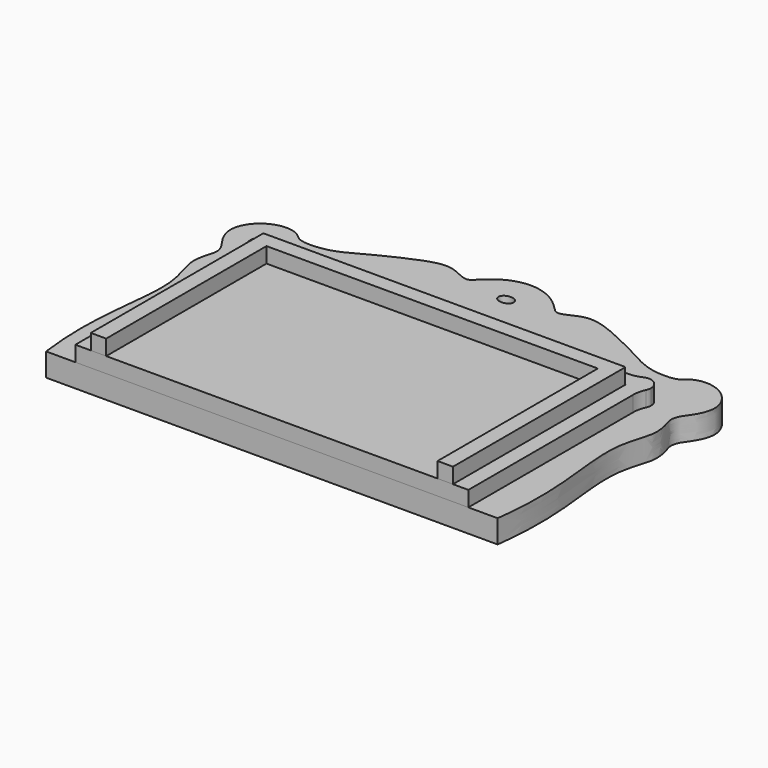
from build123d import *

# Parameters (mm, degrees)
F3_DEPTH  = 15
F5_DEPTH  = 10
F6_R      = 20
F8_DEPTH  = 10
F9_W      = 215
F9_H      = 130
F10_DEPTH = 10


# Not quite as in the source:
# - a feature names something its author has since deleted; it is built from what else it names


with BuildPart() as f3:
    # F2 (on offset) → F3 (new body)
    with BuildSketch(Plane.XY.offset(100)):
        with BuildLine():
            add(Edge.make_bspline(
                [(-146.497, 0), (-149.5984924285, 24.1158641447), (-148.0861706874, 57.3285451295), (-141.9737942158, 98.5465216918), (-150.8716245384, 120.1352309784), (-150.0828583406, 127.8333799004), (-149.2091995607, 133.0357574413), (-146.7644359487, 138.969514697), (-148.7060186985, 145.4416060002), (-153.4320405507, 150.8180485227), (-159.2044434643, 163.229297572), (-152.2232789146, 177.3369452319), (-138.5120912335, 183.3796622376), (-127.657061459, 180.8243319765), (-123.7549340061, 175.7598872143), (-115.4966109213, 174.5749138288), (-101.1868476342, 175.8719474345), (-83.9780063011, 186.2524528593), (-68.1221038647, 193.6100878861), (-57.6143130787, 198.1949467154), (-46.4912789312, 200.9893875839), (-38.3855377787, 198.1650207363), (-34.3252044535, 195.9531038256), (-28.5769681871, 194.0801714579), (-24.8215233637, 198.3952390386), (-15.2356704617, 207.2522812764), (0, 211.4399134414), (15.2356704617, 207.2522812764), (24.8215233637, 198.3952390386), (28.5769681871, 194.0801714579), (34.3252044535, 195.9531038256), (38.3855377787, 198.1650207363), (46.4912789312, 200.9893875839), (57.6143130787, 198.1949467154), (68.1221038647, 193.6100878861), (83.9780063011, 186.2524528593), (101.1868476342, 175.8719474345), (115.4966109213, 174.5749138288), (123.7549340061, 175.7598872143), (127.657061459, 180.8243319765), (138.5120912335, 183.3796622376), (152.2232789146, 177.3369452319), (159.2044434643, 163.229297572), (153.4320405507, 150.8180485227), (148.7060186985, 145.4416060002), (146.7644359487, 138.969514697), (149.2091995607, 133.0357574413), (150.0828583406, 127.8333799004), (150.8716245384, 120.1352309784), (141.9737942158, 98.5465216918), (148.0861706874, 57.3285451295), (149.5984924285, 24.1158641447), (146.497, 0)],
                knots=[0, 0, 0, 0, 0.0445117001, 0.0808774056, 0.107575939, 0.1227793119, 0.1357551155, 0.1500456603, 0.1643362052, 0.1797671231, 0.2002043009, 0.2219477978, 0.2436912948, 0.2620418522, 0.2758571435, 0.2916470183, 0.3132257177, 0.3392061483, 0.3632884541, 0.3827866647, 0.4019539182, 0.4183166408, 0.4309215947, 0.4439460967, 0.456795292, 0.4773590218, 0.5, 0.5226409782, 0.543204708, 0.5560539033, 0.5690784053, 0.5816833592, 0.5980460818, 0.6172133353, 0.6367115459, 0.6607938517, 0.6867742823, 0.7083529817, 0.7241428565, 0.7379581478, 0.7563087052, 0.7780522022, 0.7997956991, 0.8202328769, 0.8356637948, 0.8499543397, 0.8642448845, 0.8772206881, 0.892424061, 0.9191225944, 0.9554882999, 1, 1, 1, 1], degree=3))
            Line((-146.497, 0), (146.497, 0))
        make_face()
        with BuildLine():
            add(Edge.make_bspline(
                [(5, 190), (5, 196.4951905284), (-2.5, 193.2475952642), (-10, 190), (-2.5, 186.7524047358), (5, 183.5048094716), (5, 190)],
                knots=[0, 0, 0, 2.0943951024, 2.0943951024, 4.1887902048, 4.1887902048, 6.2831853072, 6.2831853072, 6.2831853072], degree=2, weights=[1, 0.5, 1, 0.5, 1, 0.5, 1]))
        make_face(mode=Mode.SUBTRACT)
    extrude(amount=F3_DEPTH)


with BuildPart() as f5:
    # F4 (on face) → F5 (new body)
    with BuildSketch(Plane.XY.offset(115)):
        with BuildLine():
            Line((-116.9098300563, 150), (-127.5, 150))
            Line((-127.5, 150), (-117.5, 140))
            Line((-117.5, 140), (-116.9098300563, 140))
            ThreePointArc((-116.9098300563, 140), (-115.4937073078, 142.3238343267), (-115, 145))
            ThreePointArc((-115, 145), (-115.4937073078, 147.6761656733), (-116.9098300563, 150))
        make_face()
        with BuildLine():
            Line((116.9098300563, 150), (-116.9098300563, 150))
            ThreePointArc((-116.9098300563, 150), (-115.4937073078, 147.6761656733), (-115, 145))
            ThreePointArc((-115, 145), (-115.4937073078, 142.3238343267), (-116.9098300563, 140))
            Line((-116.9098300563, 140), (116.9098300563, 140))
            ThreePointArc((116.9098300563, 140), (115, 145), (116.9098300563, 150))
        make_face()
        with BuildLine():
            Line((117.5, 140), (117.5, 139.4098300563))
            ThreePointArc((117.5, 139.4098300563), (122.5, 137.5), (127.5, 139.4098300563))
            Line((127.5, 139.4098300563), (127.5, 150))
            Line((127.5, 150), (116.9098300563, 150))
            ThreePointArc((116.9098300563, 150), (115, 145), (116.9098300563, 140))
            Line((116.9098300563, 140), (117.5, 140))
        make_face()
        with BuildLine():
            Line((-117.5, 139.4098300563), (-117.5, 0))
            Line((-117.5, 0), (117.5, 0))
            Line((117.5, 0), (117.5, 139.4098300563))
            ThreePointArc((117.5, 139.4098300563), (117.1966991411, 139.6966991411), (116.9098300563, 140))
            Line((116.9098300563, 140), (-116.9098300563, 140))
            ThreePointArc((-116.9098300563, 140), (-117.1966991411, 139.6966991411), (-117.5, 139.4098300563))
        make_face()
        with BuildLine():
            Line((-127.5, 150), (-127.5, 139.4098300563))
            ThreePointArc((-127.5, 139.4098300563), (-122.5, 137.5), (-117.5, 139.4098300563))
            Line((-117.5, 139.4098300563), (-117.5, 140))
            Line((-117.5, 140), (-127.5, 150))
        make_face()
        with BuildLine():
            Line((-117.5, 140), (-117.5, 139.4098300563))
            ThreePointArc((-117.5, 139.4098300563), (-117.1966991411, 139.6966991411), (-116.9098300563, 140))
            Line((-116.9098300563, 140), (-117.5, 140))
        make_face()
        with BuildLine():
            Line((-127.5, 139.4098300563), (-127.5, 0))
            Line((-127.5, 0), (-117.5, 0))
            Line((-117.5, 0), (-117.5, 139.4098300563))
            ThreePointArc((-117.5, 139.4098300563), (-122.5, 137.5), (-127.5, 139.4098300563))
        make_face()
        with BuildLine():
            Line((117.5, 139.4098300563), (117.5, 0))
            Line((117.5, 0), (127.5, 0))
            Line((127.5, 0), (127.5, 139.4098300563))
            ThreePointArc((127.5, 139.4098300563), (122.5, 137.5), (117.5, 139.4098300563))
        make_face()
        with BuildLine():
            ThreePointArc((-116.9098300563, 150), (-127.8033008589, 150.3033008589), (-127.5, 139.4098300563))
            Line((-127.5, 139.4098300563), (-127.5, 150))
            Line((-127.5, 150), (-116.9098300563, 150))
        make_face()
        with BuildLine():
            ThreePointArc((130, 145), (125.1761656733, 152.0062926922), (116.9098300563, 150))
            Line((116.9098300563, 150), (127.5, 150))
            Line((127.5, 150), (127.5, 139.4098300563))
            ThreePointArc((127.5, 139.4098300563), (129.3465319688, 141.9381378215), (130, 145))
        make_face()
    extrude(amount=F5_DEPTH)

    # F6
    f6_edges = [f5.edges().sort_by_distance(p)[0] for p in [
        (-116.90983, 150, 120),
        (-127.5, 139.40983, 120),
        (116.90983, 150, 120),
        (127.5, 139.40983, 120),
    ]]
    fillet(f6_edges, radius=F6_R)


with BuildPart() as f8:
    # F7 (on face) → F8 (new body)
    with BuildSketch(Plane.XY.offset(125)):
        with BuildLine():
            Line((-117.5, 0), (117.5, 0))
            Line((117.5, 0), (117.5, 139.4098300563))
            ThreePointArc((117.5, 139.4098300563), (117.1966991411, 139.6966991411), (116.9098300563, 140))
            Line((116.9098300563, 140), (-117.5, 140))
            Line((-117.5, 140), (-117.5, 0))
        make_face()
    extrude(amount=F8_DEPTH)

    # F9 (on face) → F10 (cut)
    with BuildSketch(Plane.XY.offset(135)):
        with Locations((0, 65)):
            Rectangle(F9_W, F9_H)
    extrude(amount=-F10_DEPTH, mode=Mode.SUBTRACT)


solid = Compound([f3.part, f5.part, f8.part])
